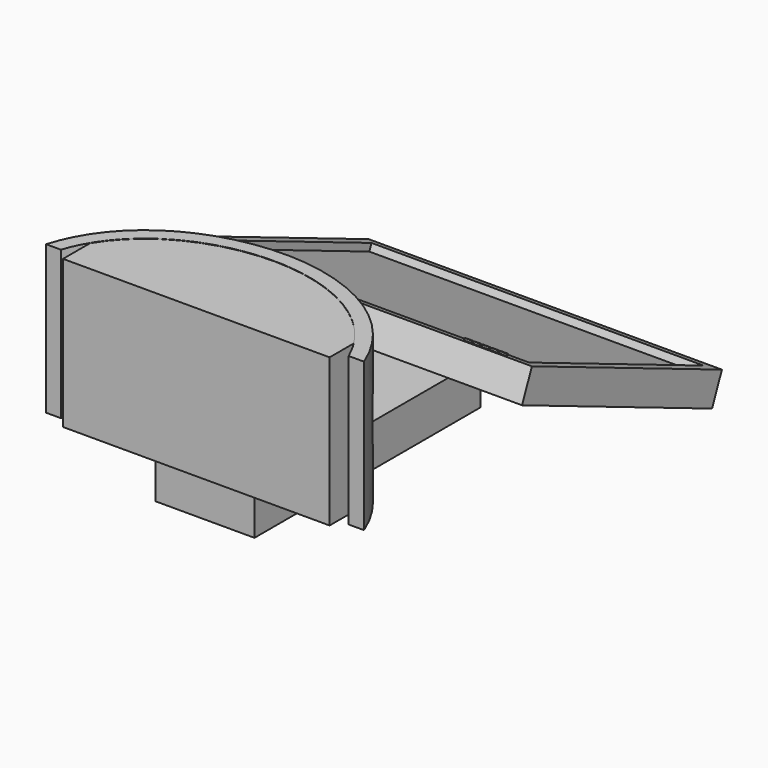
from build123d import *

# Parameters (mm, degrees)
F1_DEPTH  = 42
F2_W      = 75.478619273
F2_H      = 41.9138409197
F4_W      = 75.478619273
F4_H      = 41.9138409197
F5_DEPTH  = 3
F6_W      = 28
F6_H      = 12
F8_DEPTH  = 80
F11_W     = 100
F11_H     = 72.9077620213
F12_DEPTH = 7
F13_W     = 100
F13_H     = 72.9077620213
F13_W_2   = 94
F13_H_2   = 66.9077620213
F14_DEPTH = 2
F15_W     = 2
F15_H     = 0.5
F16_DEPTH = 0.5


# Not quite as in the source:
# - ends of sketch curves that miss each other by under 0.0002 mm in the source are joined
# - the dataset's text gives a spline's control points without its knots; the knots are read off the source's solid


with BuildPart() as f1:
    # F0 (on Top) → F1 (new body)
    with BuildSketch(Plane.XY):
        with BuildLine():
            Line((40.6705020705, 0), (45, 0))
            add(Edge.make_bspline(
                [(45, 0), (37.6566936716, 18.7177697445), (0.7563031661, 39.2432392178), (-39.1693000037, 19.753647335), (-45, 0)],
                knots=[0, 0, 0, 0, 0.5, 1, 1, 1, 1], degree=3))
            Line((-45, 0), (-40.8081785045, 0))
            add(Edge.make_bspline(
                [(40.6705020705, 0), (39.0654786869, 3.6685119371), (34.6366166878, 10.6499395063), (25.1941828283, 18.6625093529), (13.2155095249, 23.898149118), (2.1979882903, 25.5001155824), (-6.7612672319, 25.0396744323), (-15.5822493226, 23.419843787), (-23.8190972997, 20.0776830737), (-30.7940742115, 15.0930436532), (-35.2531784066, 10.5526098036), (-38.6097824931, 5.5150177421), (-40.2124471126, 1.7897260912), (-40.8081785045, 0)],
                knots=[0.0144696894, 0.0144696894, 0.0144696894, 0.0144696894, 0.125, 0.25, 0.375, 0.5, 0.5625, 0.625, 0.75, 0.8125, 0.875, 0.9375, 0.989221235, 0.989221235, 0.989221235, 0.989221235], degree=3))
        make_face()
    extrude(amount=F1_DEPTH)

    # F2 (on Front) → F3 (join, up to the next surface of F1)
    with BuildSketch(Plane.XZ):
        with Locations((-0.0689039235, 20.9569204599)):
            Rectangle(F2_W, F2_H)
    extrude(until=Until.NEXT, dir=(0, 1, 0))

    # F4 (on face) → F5 (join)
    with BuildSketch(Plane.XZ):
        with Locations((-0.0689039235, 20.9569204599)):
            Rectangle(F4_W, F4_H)
    extrude(amount=F5_DEPTH)

    # F6 (on Front) → F8 (join)
    with BuildSketch(Plane.XZ):
        with Locations((0, -6)):
            Rectangle(F6_W, F6_H)
    extrude(amount=-F8_DEPTH)

    # F11 (on face) → F12 (join)
    with BuildSketch(Plane(origin=(0, 11.8870032706, 28.3832509576), x_dir=(1, 0, 0), z_dir=(0, 0.3862941051, 0.9223756634))):
        with Locations((0, 77.4465687573)):
            Rectangle(F11_W, F11_H)
    extrude(amount=F12_DEPTH)

    # F13 (on face) → F14 (join)
    with BuildSketch(Plane(origin=(0, 14.591062006, 34.8398806013), x_dir=(1, 0, 0), z_dir=(0, 0.3862941051, 0.9223756634))):
        with Locations((0, 77.4465687573)):
            Rectangle(F13_W, F13_H)
        with Locations((0, 77.4465687573)):
            Rectangle(F13_W_2, F13_H_2, mode=Mode.SUBTRACT)
    extrude(amount=F14_DEPTH)

    # F15 (on face) → F16 (join)
    with BuildSketch(Plane(origin=(0, 15.3636502161, 36.684631928), x_dir=(1, 0, 0), z_dir=(0, 0.3862941051, 0.9223756634))):
        with Locations((33.4735295493, 42.3066589715)):
            Rectangle(F15_W, F15_H)
        with Locations((35.9735295493, 42.3066589715)):
            Rectangle(F15_W, F15_H)
        with Locations((38.4735295493, 42.3066589715)):
            Rectangle(F15_W, F15_H)
        with Locations((40.9735295493, 42.3066589715)):
            Rectangle(F15_W, F15_H)
        with Locations((30.9735295493, 42.3066589715)):
            Rectangle(F15_W, F15_H)
    extrude(amount=F16_DEPTH)


solid = f1.part
